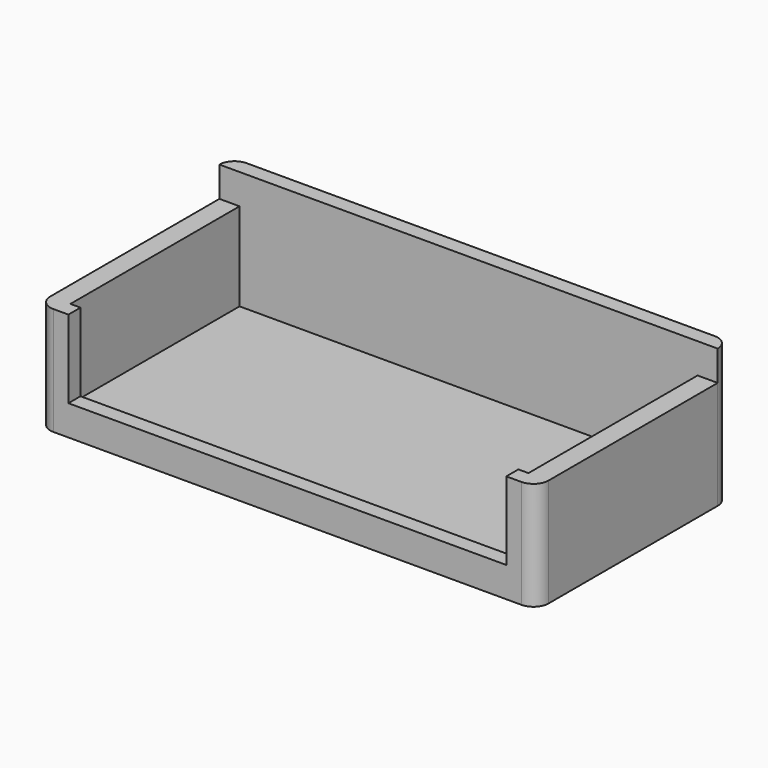
from build123d import *

# Parameters (mm, degrees)
F0_W     = 99
F0_H     = 6
F1_DEPTH = 48
F3_DEPTH = 15.5
F4_W     = 2
F4_H     = 42
F4_W_2   = 87
F5_DEPTH = 17.5
F6_DEPTH = 6
F7_R     = 2.99999


# Not quite as in the source:
# - a fillet or chamfer is up to 0.001 mm smaller than in the source, because OpenCascade refuses the exact size


with BuildPart() as f1:
    # F0 (on Front) → F1 (new body)
    with BuildSketch(Plane.XZ):
        with Locations((0, 3)):
            Rectangle(F0_W, F0_H)
    extrude(amount=F1_DEPTH)

    # F2 (on face) → F3 (join)
    with BuildSketch(Plane.XY.offset(6)):
        Polygon((49.5, -3), (49.5, 0), (43.5, 0), (-43.5, 0), (-49.5, 0), (-49.5, -3), (-49.5, -48), (-43.5, -48), (-43.5, -3), (43.5, -3), (43.5, -48), (49.5, -48), align=None)
    extrude(amount=F3_DEPTH)

    # F4 (on face) → F5 (cut)
    with BuildSketch(Plane.XY.offset(21.5)):
        with Locations((-44.5, -24)):
            Rectangle(F4_W, F4_H)
        with Locations((0, -24)):
            Rectangle(F4_W_2, F4_H)
        with Locations((44.5, -24)):
            Rectangle(F4_W, F4_H)
    extrude(amount=-F5_DEPTH, mode=Mode.SUBTRACT)

    # F4 (on face) → F6 (join)
    with BuildSketch(Plane.XY.offset(21.5)):
        Polygon((-49.5, -3), (-45.5, -3), (-43.5, -3), (43.5, -3), (45.5, -3), (49.5, -3), (49.5, 0), (-49.5, 0), align=None)
    extrude(amount=F6_DEPTH)

    # F7 (radius 3 in the source; OpenCascade refuses exactly that, so slightly less here)
    f7_edges = [f1.edges().sort_by_distance(p)[0] for p in [
        (-49.5, -48, 10.75),
        (49.5, -48, 10.75),
        (49.5, 0, 13.75),
        (-49.5, 0, 13.75),
    ]]
    fillet(f7_edges, radius=F7_R)


solid = f1.part
